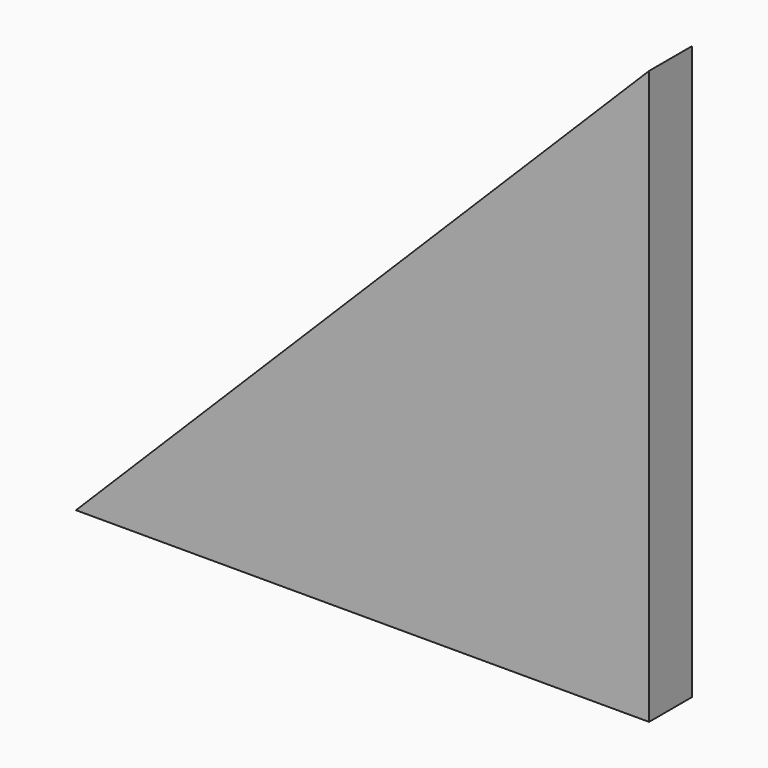
from build123d import *

# Parameters (mm, degrees)
F1_DEPTH = 4.7625


# Not quite as in the source:
# - a length typed as a fraction of an inch, garbled in the dataset ("3 / 203.2 mm" for 3/8 in), is restored


with BuildPart() as f1:
    # F0 (on Front) → F1 (new body)
    with BuildSketch(Plane.XZ):
        Polygon((50.8, 50.8), (0, 0), (50.8, 0), align=None)
    extrude(amount=F1_DEPTH)


solid = f1.part
